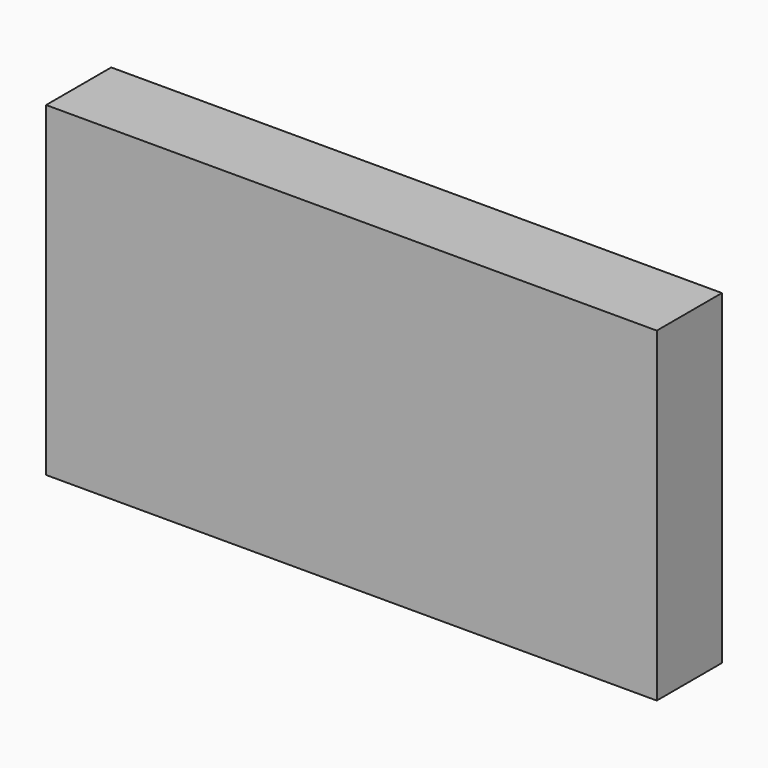
from build123d import *

# Parameters (mm, degrees)
F0_W     = 2.5
F0_H     = 17
F1_DEPTH = 10
F2_DEPTH = 7.5


# Not quite as in the source:
# - a feature names something its author has since deleted; it is built from what else it names


with BuildPart() as f1:
    # F0 (on Front) → F1 (new body)
    with BuildSketch(Plane.XZ):
        Polygon((37.5, 20), (-37.5, 20), (-37.5, 10.2), (-35, 10.2), (-35, 17.5), (35, 17.5), (35, -17.5), (-35, -17.5), (-35, -6.8), (-37.5, -6.8), (-37.5, -20), (37.5, -20), align=None)
        with Locations((-36.25, 1.7)):
            Rectangle(F0_W, F0_H)
        Polygon((-35, 17.5), (-35, 10.2), (-35, -6.8), (-35, -17.5), (35, -17.5), (35, 17.5), align=None)
    extrude(amount=F1_DEPTH)

    # F0 (on Front) → F2 (cut)
    with BuildSketch(Plane.XZ):
        Polygon((-35, 17.5), (-35, 10.2), (-35, -6.8), (-35, -17.5), (35, -17.5), (35, 17.5), align=None)
        with Locations((-36.25, 1.7)):
            Rectangle(F0_W, F0_H)
    extrude(amount=F2_DEPTH, mode=Mode.SUBTRACT)


solid = f1.part
